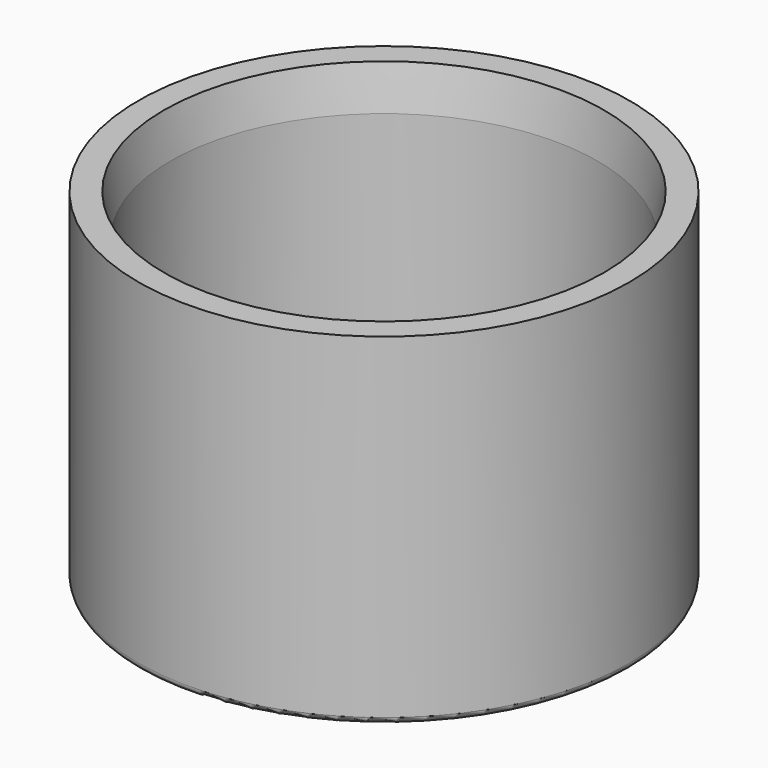
from build123d import *

# Parameters (mm, degrees)
F2_R     = 11.5
F2_R_2   = 10
F3_DEPTH = 16
F4_DEPTH = 1.5
F5_R     = 0.3
F6_SIZE2 = 0.3
F6_SIZE  = 2


with BuildPart() as f3:
    # F2 (on Top) → F3 (new body)
    with BuildSketch(Plane.XY):
        Circle(F2_R)
        Circle(F2_R_2, mode=Mode.SUBTRACT)
    extrude(amount=F3_DEPTH)

    # F2 (on Top) → F4 (join)
    with BuildSketch(Plane.XY):
        Circle(F2_R_2)
    extrude(amount=F4_DEPTH)

    # F5
    f5_edges = [f3.edges().sort_by_distance(p)[0] for p in [
        (-11.5, 0, 0),
    ]]
    fillet(f5_edges, radius=F5_R)

    # F6
    f6_edges = [f3.edges().sort_by_distance(p)[0] for p in [
        (-10, 0, 16),
    ]]
    f6_side = f3.faces().sort_by_distance((-10, 0, 8.75))[0]
    chamfer(f6_edges, length=F6_SIZE, length2=F6_SIZE2, reference=f6_side)


solid = f3.part
